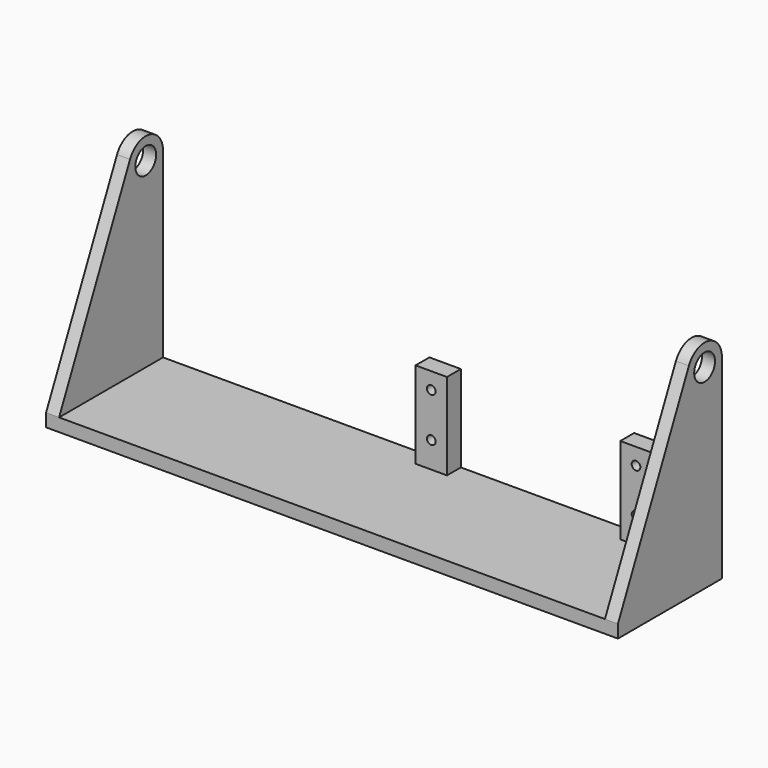
from build123d import *

# Parameters (mm, degrees)
F0_W     = 126
F0_H     = 30
F1_DEPTH = 3
F2_R     = 3
F2_W     = 30
F2_H     = 3
F3_DEPTH = 3
F4_W     = 7.26
F4_H     = 4
F5_DEPTH = 20
F6_R     = 1
F7_DEPTH = 4


# Not quite as in the source:
# - a pattern or mirror of a feature is missing from the dataset's text; its kind, count and spacing are read off the source's solid


with BuildPart() as f1:
    # F0 (on Top) → F1 (new body)
    with BuildSketch(Plane.XY):
        Rectangle(F0_W, F0_H)
    extrude(amount=F1_DEPTH)

    # F2 (on face) → F3 (join)
    with BuildSketch(Plane.YZ.offset(63)):
        with BuildLine():
            Line((-15, 3), (15, 3))
            Line((15, 3), (15, 45))
            ThreePointArc((15, 45), (11.0775660253, 49.8825046299), (5.4644594156, 47.1044884431))
            Line((5.4644594156, 47.1044884431), (-15, 3))
        make_face()
        with Locations((10, 45)):
            Circle(F2_R, mode=Mode.SUBTRACT)
        with Locations((0, 1.5)):
            Rectangle(F2_W, F2_H)
    f3 = extrude(amount=F3_DEPTH)

    # F3_copies: F3 across plane
    add(f3.mirror(Plane(origin=(0, 0, 0), x_dir=(0, 0, -1), z_dir=(-1, 0, 0))))

    # F4 (on face) → F5 (join)
    with BuildSketch(Plane.XY.offset(3)):
        with Locations((2.11, 13)):
            Rectangle(F4_W, F4_H)
        with Locations((49.37, 13)):
            Rectangle(F4_W, F4_H)
    extrude(amount=F5_DEPTH)

    # F6 (on face) → F7 (cut, through all)
    with BuildSketch(Plane(origin=(0, 15, 0), x_dir=(-1, 0, 0), z_dir=(0, 1, 0))):
        with Locations((-49.37, 19.17)):
            Circle(F6_R)
        with Locations((-49.37, 9)):
            Circle(F6_R)
        with Locations((-2.11, 19.17)):
            Circle(F6_R)
        with Locations((-2.11, 9)):
            Circle(F6_R)
    extrude(amount=-F7_DEPTH, mode=Mode.SUBTRACT)


solid = f1.part
